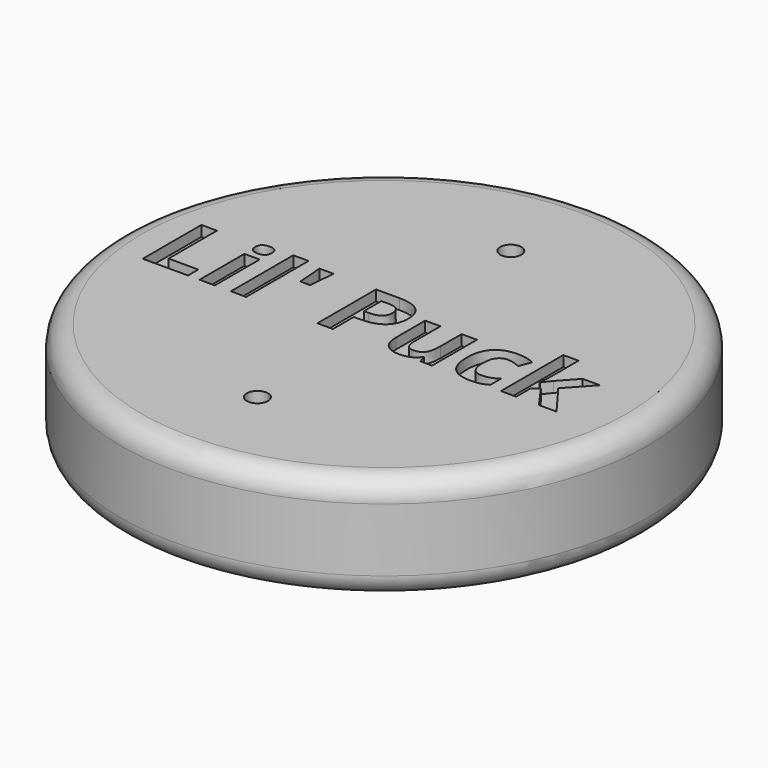
from build123d import *

# Parameters (mm, degrees)
F0_R           = 25
F1_DEPTH       = 10
F2_TEXT_SIZE   = 9.7222222222
F3_DEPTH       = 1
F4_R           = 2
F6_D           = 2
F6_CBORE_D     = 5
F6_CBORE_DEPTH = 2.5


# Not quite as in the source:
# - Text() gives the source's letters only with a copy of the font that has no kerning and outlines rounded to 1/6400 em; it was checked with that copy


with BuildPart() as f1:
    # F0 (on Top) → F1 (new body)
    with BuildSketch(Plane.XY):
        Circle(F0_R)
    extrude(amount=F1_DEPTH)

    # F2 (on face) → F3 (cut)
    with BuildSketch(Plane.XY.offset(10)):
        with Locations((-21.3389738566, -2.9905730882)):
            Text("Lil' Puck", F2_TEXT_SIZE, font='Open Sans', font_style=FontStyle.BOLD, text_align=(TextAlign.LEFT, TextAlign.BOTTOM))
    extrude(amount=-F3_DEPTH, mode=Mode.SUBTRACT)

    # F4
    f4_edges = [f1.edges().sort_by_distance(p)[0] for p in [
        (-25, 0, 10),
        (-25, 0, 0),
    ]]
    fillet(f4_edges, radius=F4_R)

    # F6 (through all)
    with Locations(Plane(origin=(0, 0, 0), x_dir=(1, 0, 0), z_dir=(0, 0, -1))):
        with Locations((0, 15), (0, -15)):
            CounterBoreHole(F6_D / 2, F6_CBORE_D / 2, F6_CBORE_DEPTH)


solid = f1.part
